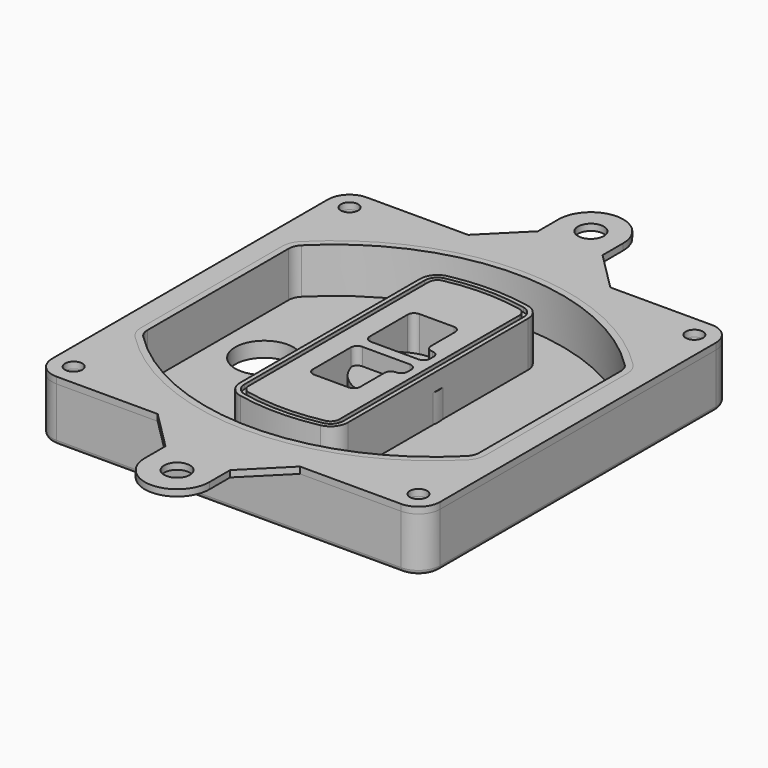
from build123d import *

# Parameters (mm, degrees)
F0_R      = 4
F1_DEPTH  = 25
F2_DEPTH  = 3
F3_DEPTH  = 18
F5_DEPTH  = 21
F6_DEPTH  = 2
F8_DEPTH  = 20
F9_DEPTH  = 16
F10_DEPTH = 25
F7_R      = 6
F7_R_2    = 4
F11_DEPTH = 6
F13_DEPTH = 9
F15_R     = 2
F16_R     = 4
F16_R_2   = 6
F17_DEPTH = 3


# Not quite as in the source:
# - a feature of the source that left no trace in its solid (it failed there, or was rolled back) is left out
# - a feature names something its author has since deleted; it is built from what else it names


with BuildPart() as f1:
    # F0 (on Top) → F1 (new body)
    with BuildSketch(Plane.XY):
        with BuildLine():
            ThreePointArc((-90, -80), (-87.0710678119, -87.0710678119), (-80, -90))
            Line((-80, -90), (80, -90))
            ThreePointArc((80, -90), (87.0710678119, -87.0710678119), (90, -80))
            Line((90, -80), (90, 80))
            ThreePointArc((90, 80), (87.0710678119, 87.0710678119), (80, 90))
            Line((80, 90), (-80, 90))
            ThreePointArc((-80, 90), (-87.0710678119, 87.0710678119), (-90, 80))
            Line((-90, 80), (-90, -80))
        make_face()
        with Locations((-80, -80)):
            Circle(F0_R, mode=Mode.SUBTRACT)
        with Locations((80, -80)):
            Circle(F0_R, mode=Mode.SUBTRACT)
        with BuildLine():
            ThreePointArc((-84, 40.977524478), (-82.9361107095, 46.3307515151), (-79.9061371841, 50.8703727074))
            ThreePointArc((-79.9061371841, 50.8703727074), (0, 84), (79.9061371841, 50.8703727074))
            ThreePointArc((79.9061371841, 50.8703727074), (82.9361107095, 46.3307515151), (84, 40.977524478))
            Line((84, 40.977524478), (84, -40.977524478))
            ThreePointArc((84, -40.977524478), (82.9361107095, -46.3307515151), (79.9061371841, -50.8703727074))
            ThreePointArc((79.9061371841, -50.8703727074), (0, -84), (-79.9061371841, -50.8703727074))
            ThreePointArc((-79.9061371841, -50.8703727074), (-82.9361107095, -46.3307515151), (-84, -40.977524478))
            Line((-84, -40.977524478), (-84, 40.977524478))
        make_face(mode=Mode.SUBTRACT)
        with Locations((-80, 80)):
            Circle(F0_R, mode=Mode.SUBTRACT)
        with Locations((80, 80)):
            Circle(F0_R, mode=Mode.SUBTRACT)
        with BuildLine():
            ThreePointArc((79.9061371841, 50.8703727074), (0, 84), (-79.9061371841, 50.8703727074))
            ThreePointArc((-79.9061371841, 50.8703727074), (-82.9361107095, 46.3307515151), (-84, 40.977524478))
            Line((-84, 40.977524478), (-84, -40.977524478))
            ThreePointArc((-84, -40.977524478), (-82.9361107095, -46.3307515151), (-79.9061371841, -50.8703727074))
            ThreePointArc((-79.9061371841, -50.8703727074), (0, -84), (79.9061371841, -50.8703727074))
            ThreePointArc((79.9061371841, -50.8703727074), (82.9361107095, -46.3307515151), (84, -40.977524478))
            Line((84, -40.977524478), (84, 40.977524478))
            ThreePointArc((84, 40.977524478), (82.9361107095, 46.3307515151), (79.9061371841, 50.8703727074))
        make_face()
        with BuildLine():
            Line((-80, -40.977524478), (-80, 40.977524478))
            ThreePointArc((-80, 40.977524478), (-79.2400790782, 44.801258076), (-77.0758122744, 48.0438446418))
            ThreePointArc((-77.0758122744, 48.0438446418), (0, 80), (77.0758122744, 48.0438446418))
            ThreePointArc((77.0758122744, 48.0438446418), (79.2400790782, 44.801258076), (80, 40.977524478))
            Line((80, 40.977524478), (80, -40.977524478))
            ThreePointArc((80, -40.977524478), (79.2400790782, -44.801258076), (77.0758122744, -48.0438446418))
            ThreePointArc((77.0758122744, -48.0438446418), (0, -80), (-77.0758122744, -48.0438446418))
            ThreePointArc((-77.0758122744, -48.0438446418), (-79.2400790782, -44.801258076), (-80, -40.977524478))
        make_face(mode=Mode.SUBTRACT)
        with BuildLine():
            ThreePointArc((-77.0758122744, 48.0438446418), (-79.2400790782, 44.801258076), (-80, 40.977524478))
            Line((-80, 40.977524478), (-80, -40.977524478))
            ThreePointArc((-80, -40.977524478), (-79.2400790782, -44.801258076), (-77.0758122744, -48.0438446418))
            ThreePointArc((-77.0758122744, -48.0438446418), (0, -80), (77.0758122744, -48.0438446418))
            ThreePointArc((77.0758122744, -48.0438446418), (79.2400790782, -44.801258076), (80, -40.977524478))
            Line((80, -40.977524478), (80, 40.977524478))
            ThreePointArc((80, 40.977524478), (79.2400790782, 44.801258076), (77.0758122744, 48.0438446418))
            ThreePointArc((77.0758122744, 48.0438446418), (0, 80), (-77.0758122744, 48.0438446418))
        make_face()
        with BuildLine():
            ThreePointArc((74.9530685921, 45.9239485927), (76.4680553548, 43.6541379966), (77, 40.977524478))
            Line((77, 40.977524478), (77, -40.977524478))
            ThreePointArc((77, -40.977524478), (76.4680553548, -43.6541379966), (74.9530685921, -45.9239485927))
            ThreePointArc((74.9530685921, -45.9239485927), (0, -77), (-74.9530685921, -45.9239485927))
            ThreePointArc((-74.9530685921, -45.9239485927), (-76.4680553548, -43.6541379966), (-77, -40.977524478))
            Line((-77, -40.977524478), (-77, 40.977524478))
            ThreePointArc((-77, 40.977524478), (-76.4680553548, 43.6541379966), (-74.9530685921, 45.9239485927))
            ThreePointArc((-74.9530685921, 45.9239485927), (0, 77), (74.9530685921, 45.9239485927))
        make_face(mode=Mode.SUBTRACT)
        with BuildLine():
            Line((77, -40.977524478), (77, 40.977524478))
            ThreePointArc((77, 40.977524478), (76.4680553548, 43.6541379966), (74.9530685921, 45.9239485927))
            ThreePointArc((74.9530685921, 45.9239485927), (0, 77), (-74.9530685921, 45.9239485927))
            ThreePointArc((-74.9530685921, 45.9239485927), (-76.4680553548, 43.6541379966), (-77, 40.977524478))
            Line((-77, 40.977524478), (-77, -40.977524478))
            ThreePointArc((-77, -40.977524478), (-76.4680553548, -43.6541379966), (-74.9530685921, -45.9239485927))
            ThreePointArc((-74.9530685921, -45.9239485927), (0, -77), (74.9530685921, -45.9239485927))
            ThreePointArc((74.9530685921, -45.9239485927), (76.4680553548, -43.6541379966), (77, -40.977524478))
        make_face()
    extrude(amount=-F1_DEPTH)

    # F0 (on Top) → F2 (join)
    with BuildSketch(Plane.XY):
        with BuildLine():
            ThreePointArc((-77.0758122744, 48.0438446418), (-79.2400790782, 44.801258076), (-80, 40.977524478))
            Line((-80, 40.977524478), (-80, -40.977524478))
            ThreePointArc((-80, -40.977524478), (-79.2400790782, -44.801258076), (-77.0758122744, -48.0438446418))
            ThreePointArc((-77.0758122744, -48.0438446418), (0, -80), (77.0758122744, -48.0438446418))
            ThreePointArc((77.0758122744, -48.0438446418), (79.2400790782, -44.801258076), (80, -40.977524478))
            Line((80, -40.977524478), (80, 40.977524478))
            ThreePointArc((80, 40.977524478), (79.2400790782, 44.801258076), (77.0758122744, 48.0438446418))
            ThreePointArc((77.0758122744, 48.0438446418), (0, 80), (-77.0758122744, 48.0438446418))
        make_face()
        with BuildLine():
            ThreePointArc((74.9530685921, 45.9239485927), (76.4680553548, 43.6541379966), (77, 40.977524478))
            Line((77, 40.977524478), (77, -40.977524478))
            ThreePointArc((77, -40.977524478), (76.4680553548, -43.6541379966), (74.9530685921, -45.9239485927))
            ThreePointArc((74.9530685921, -45.9239485927), (0, -77), (-74.9530685921, -45.9239485927))
            ThreePointArc((-74.9530685921, -45.9239485927), (-76.4680553548, -43.6541379966), (-77, -40.977524478))
            Line((-77, -40.977524478), (-77, 40.977524478))
            ThreePointArc((-77, 40.977524478), (-76.4680553548, 43.6541379966), (-74.9530685921, 45.9239485927))
            ThreePointArc((-74.9530685921, 45.9239485927), (0, 77), (74.9530685921, 45.9239485927))
        make_face(mode=Mode.SUBTRACT)
    extrude(amount=F2_DEPTH)

    # F0 (on Top) → F3 (cut)
    with BuildSketch(Plane.XY):
        with BuildLine():
            Line((77, -40.977524478), (77, 40.977524478))
            ThreePointArc((77, 40.977524478), (76.4680553548, 43.6541379966), (74.9530685921, 45.9239485927))
            ThreePointArc((74.9530685921, 45.9239485927), (0, 77), (-74.9530685921, 45.9239485927))
            ThreePointArc((-74.9530685921, 45.9239485927), (-76.4680553548, 43.6541379966), (-77, 40.977524478))
            Line((-77, 40.977524478), (-77, -40.977524478))
            ThreePointArc((-77, -40.977524478), (-76.4680553548, -43.6541379966), (-74.9530685921, -45.9239485927))
            ThreePointArc((-74.9530685921, -45.9239485927), (0, -77), (74.9530685921, -45.9239485927))
            ThreePointArc((74.9530685921, -45.9239485927), (76.4680553548, -43.6541379966), (77, -40.977524478))
        make_face()
    extrude(amount=-F3_DEPTH, mode=Mode.SUBTRACT)

    # F4 (on face) → F5 (join, through all)
    with BuildSketch(Plane.XY.offset(3)):
        with BuildLine():
            ThreePointArc((-25, -52.2388355719), (-23.2096587819, -57.2826573186), (-18.6399655469, -60.0689385728))
            ThreePointArc((-18.6399655469, -60.0689385728), (0, -62), (18.6399655469, -60.0689385728))
            ThreePointArc((18.6399655469, -60.0689385728), (23.2096587819, -57.2826573186), (25, -52.2388355719))
            Line((25, -52.2388355719), (25, 52.2388355719))
            ThreePointArc((25, 52.2388355719), (23.2096587819, 57.2826573186), (18.6399655469, 60.0689385728))
            ThreePointArc((18.6399655469, 60.0689385728), (0, 62), (-18.6399655469, 60.0689385728))
            ThreePointArc((-18.6399655469, 60.0689385728), (-23.2096587819, 57.2826573186), (-25, 52.2388355719))
            Line((-25, 52.2388355719), (-25, -52.2388355719))
        make_face()
        with BuildLine():
            ThreePointArc((18.2299741602, 58.1114128226), (21.6572440864, 56.0217018819), (23, 52.2388355719))
            Line((23, 52.2388355719), (23, -52.2388355719))
            ThreePointArc((23, -52.2388355719), (21.6572440864, -56.0217018819), (18.2299741602, -58.1114128226))
            ThreePointArc((18.2299741602, -58.1114128226), (0, -60), (-18.2299741602, -58.1114128226))
            ThreePointArc((-18.2299741602, -58.1114128226), (-21.6572440864, -56.0217018819), (-23, -52.2388355719))
            Line((-23, -52.2388355719), (-23, 52.2388355719))
            ThreePointArc((-23, 52.2388355719), (-21.6572440864, 56.0217018819), (-18.2299741602, 58.1114128226))
            ThreePointArc((-18.2299741602, 58.1114128226), (0, 60), (18.2299741602, 58.1114128226))
        make_face(mode=Mode.SUBTRACT)
        with BuildLine():
            Line((23, -52.2388355719), (23, 52.2388355719))
            ThreePointArc((23, 52.2388355719), (21.6572440864, 56.0217018819), (18.2299741602, 58.1114128226))
            ThreePointArc((18.2299741602, 58.1114128226), (0, 60), (-18.2299741602, 58.1114128226))
            ThreePointArc((-18.2299741602, 58.1114128226), (-21.6572440864, 56.0217018819), (-23, 52.2388355719))
            Line((-23, 52.2388355719), (-23, -52.2388355719))
            ThreePointArc((-23, -52.2388355719), (-21.6572440864, -56.0217018819), (-18.2299741602, -58.1114128226))
            ThreePointArc((-18.2299741602, -58.1114128226), (0, -60), (18.2299741602, -58.1114128226))
            ThreePointArc((18.2299741602, -58.1114128226), (21.6572440864, -56.0217018819), (23, -52.2388355719))
        make_face()
        with BuildLine():
            ThreePointArc((17.8199827735, 56.1538870724), (20.104829391, 54.7607464453), (21, 52.2388355719))
            Line((21, 52.2388355719), (21, -52.2388355719))
            ThreePointArc((21, -52.2388355719), (20.104829391, -54.7607464453), (17.8199827735, -56.1538870724))
            ThreePointArc((17.8199827735, -56.1538870724), (0, -58), (-17.8199827735, -56.1538870724))
            ThreePointArc((-17.8199827735, -56.1538870724), (-20.104829391, -54.7607464453), (-21, -52.2388355719))
            Line((-21, -52.2388355719), (-21, 52.2388355719))
            ThreePointArc((-21, 52.2388355719), (-20.104829391, 54.7607464453), (-17.8199827735, 56.1538870724))
            ThreePointArc((-17.8199827735, 56.1538870724), (0, 58), (17.8199827735, 56.1538870724))
        make_face(mode=Mode.SUBTRACT)
        with BuildLine():
            Line((21, -52.2388355719), (21, 52.2388355719))
            ThreePointArc((21, 52.2388355719), (20.104829391, 54.7607464453), (17.8199827735, 56.1538870724))
            ThreePointArc((17.8199827735, 56.1538870724), (0, 58), (-17.8199827735, 56.1538870724))
            ThreePointArc((-17.8199827735, 56.1538870724), (-20.104829391, 54.7607464453), (-21, 52.2388355719))
            Line((-21, 52.2388355719), (-21, -52.2388355719))
            ThreePointArc((-21, -52.2388355719), (-20.104829391, -54.7607464453), (-17.8199827735, -56.1538870724))
            ThreePointArc((-17.8199827735, -56.1538870724), (0, -58), (17.8199827735, -56.1538870724))
            ThreePointArc((17.8199827735, -56.1538870724), (20.104829391, -54.7607464453), (21, -52.2388355719))
        make_face()
        with BuildLine():
            Line((-8, -2.5), (14, -2.5))
            ThreePointArc((14, -2.5), (16.1213203436, -3.3786796564), (17, -5.5))
            Line((17, -5.5), (17, -7.5))
            ThreePointArc((17, -7.5), (16.1213203436, -9.6213203436), (14, -10.5))
            ThreePointArc((14, -10.5), (11.8786796564, -11.3786796564), (11, -13.5))
            Line((11, -13.5), (11, -27.5))
            ThreePointArc((11, -27.5), (10.1213203436, -29.6213203436), (8, -30.5))
            Line((8, -30.5), (-8, -30.5))
            ThreePointArc((-8, -30.5), (-10.1213203436, -29.6213203436), (-11, -27.5))
            Line((-11, -27.5), (-11, -5.5))
            ThreePointArc((-11, -5.5), (-10.1213203436, -3.3786796564), (-8, -2.5))
        make_face(mode=Mode.SUBTRACT)
        with BuildLine():
            ThreePointArc((-8, 2.5), (-10.1213203436, 3.3786796564), (-11, 5.5))
            Line((-11, 5.5), (-11, 27.5))
            ThreePointArc((-11, 27.5), (-10.1213203436, 29.6213203436), (-8, 30.5))
            Line((-8, 30.5), (8, 30.5))
            ThreePointArc((8, 30.5), (10.1213203436, 29.6213203436), (11, 27.5))
            Line((11, 27.5), (11, 13.5))
            ThreePointArc((11, 13.5), (11.8786796564, 11.3786796564), (14, 10.5))
            ThreePointArc((14, 10.5), (16.1213203436, 9.6213203436), (17, 7.5))
            Line((17, 7.5), (17, 5.5))
            ThreePointArc((17, 5.5), (16.1213203436, 3.3786796564), (14, 2.5))
            Line((14, 2.5), (-8, 2.5))
        make_face(mode=Mode.SUBTRACT)
    extrude(amount=-F5_DEPTH)

    # F4 (on face) → F6 (cut)
    with BuildSketch(Plane.XY.offset(3)):
        with BuildLine():
            Line((23, -52.2388355719), (23, 52.2388355719))
            ThreePointArc((23, 52.2388355719), (21.6572440864, 56.0217018819), (18.2299741602, 58.1114128226))
            ThreePointArc((18.2299741602, 58.1114128226), (0, 60), (-18.2299741602, 58.1114128226))
            ThreePointArc((-18.2299741602, 58.1114128226), (-21.6572440864, 56.0217018819), (-23, 52.2388355719))
            Line((-23, 52.2388355719), (-23, -52.2388355719))
            ThreePointArc((-23, -52.2388355719), (-21.6572440864, -56.0217018819), (-18.2299741602, -58.1114128226))
            ThreePointArc((-18.2299741602, -58.1114128226), (0, -60), (18.2299741602, -58.1114128226))
            ThreePointArc((18.2299741602, -58.1114128226), (21.6572440864, -56.0217018819), (23, -52.2388355719))
        make_face()
        with BuildLine():
            ThreePointArc((17.8199827735, 56.1538870724), (20.104829391, 54.7607464453), (21, 52.2388355719))
            Line((21, 52.2388355719), (21, -52.2388355719))
            ThreePointArc((21, -52.2388355719), (20.104829391, -54.7607464453), (17.8199827735, -56.1538870724))
            ThreePointArc((17.8199827735, -56.1538870724), (0, -58), (-17.8199827735, -56.1538870724))
            ThreePointArc((-17.8199827735, -56.1538870724), (-20.104829391, -54.7607464453), (-21, -52.2388355719))
            Line((-21, -52.2388355719), (-21, 52.2388355719))
            ThreePointArc((-21, 52.2388355719), (-20.104829391, 54.7607464453), (-17.8199827735, 56.1538870724))
            ThreePointArc((-17.8199827735, 56.1538870724), (0, 58), (17.8199827735, 56.1538870724))
        make_face(mode=Mode.SUBTRACT)
    extrude(amount=-F6_DEPTH, mode=Mode.SUBTRACT)

    # F7 (on face) → F8 (join)
    with BuildSketch(Plane(origin=(0, 0, -25), x_dir=(1, 0, 0), z_dir=(0, 0, -1))):
        with BuildLine():
            ThreePointArc((-6.71157564, 0), (6.7567035675, 13.4682792075), (20.224982775, 0))
            Line((20.224982775, 0), (25.224982775, 0))
            ThreePointArc((25.224982775, 0), (6.7567035675, 18.4682792075), (-11.71157564, 0))
            Line((-11.71157564, 0), (-6.71157564, 0))
        make_face()
        with BuildLine():
            Line((-6.71157564, 0), (20.224982775, 0))
            ThreePointArc((20.224982775, 0), (6.7567035675, 13.4682792075), (-6.71157564, 0))
        make_face()
        with BuildLine():
            ThreePointArc((-6.71157564, 0), (6.7567035675, -13.4682792075), (20.224982775, 0))
            Line((20.224982775, 0), (-6.71157564, 0))
        make_face()
        with BuildLine():
            Line((25.224982775, 0), (20.224982775, 0))
            ThreePointArc((20.224982775, 0), (6.7567035675, -13.4682792075), (-6.71157564, 0))
            Line((-6.71157564, 0), (-11.71157564, 0))
            ThreePointArc((-11.71157564, 0), (6.7567035675, -18.4682792075), (25.224982775, 0))
        make_face()
    extrude(amount=-F8_DEPTH)

    # F7 (on face) → F9 (cut)
    with BuildSketch(Plane(origin=(0, 0, -25), x_dir=(1, 0, 0), z_dir=(0, 0, -1))):
        with BuildLine():
            Line((-6.71157564, 0), (20.224982775, 0))
            ThreePointArc((20.224982775, 0), (6.7567035675, 13.4682792075), (-6.71157564, 0))
        make_face()
        with BuildLine():
            ThreePointArc((-6.71157564, 0), (6.7567035675, -13.4682792075), (20.224982775, 0))
            Line((20.224982775, 0), (-6.71157564, 0))
        make_face()
    extrude(amount=-F9_DEPTH, mode=Mode.SUBTRACT)

    # F7 (on face) → F10 (cut)
    with BuildSketch(Plane(origin=(0, 0, -25), x_dir=(1, 0, 0), z_dir=(0, 0, -1))):
        with BuildLine():
            Line((-69.0318229325, 0), (-42.0952645175, 0))
            ThreePointArc((-42.0952645175, 0), (-55.563543725, 13.4682792075), (-69.0318229325, 0))
        make_face()
        with BuildLine():
            ThreePointArc((-69.0318229325, 0), (-55.563543725, -13.4682792075), (-42.0952645175, 0))
            Line((-42.0952645175, 0), (-69.0318229325, 0))
        make_face()
    extrude(amount=-F10_DEPTH, mode=Mode.SUBTRACT)

    # F7 (on face) → F11 (cut)
    with BuildSketch(Plane(origin=(0, 0, -25), x_dir=(1, 0, 0), z_dir=(0, 0, -1))):
        with Locations((80, -80)):
            Circle(F7_R)
        with Locations((80, -80)):
            Circle(F7_R_2, mode=Mode.SUBTRACT)
        with Locations((-80, -80)):
            Circle(F7_R)
        with Locations((-80, -80)):
            Circle(F7_R_2, mode=Mode.SUBTRACT)
        with Locations((-80, 80)):
            Circle(F7_R)
        with Locations((-80, 80)):
            Circle(F7_R_2, mode=Mode.SUBTRACT)
        with Locations((80, 80)):
            Circle(F7_R)
        with Locations((80, 80)):
            Circle(F7_R_2, mode=Mode.SUBTRACT)
    extrude(amount=-F11_DEPTH, mode=Mode.SUBTRACT)

    # F12 (on face) → F13 (cut, through all)
    with BuildSketch(Plane(origin=(0, 0, -9), x_dir=(1, 0, 0), z_dir=(0, 0, -1))):
        with BuildLine():
            ThreePointArc((20.224982775, 0), (20.1663399806, 1.2554664788), (19.9909222755, 2.5))
            Line((19.9909222755, 2.5), (14, 2.5))
            ThreePointArc((14, 2.5), (16.1213203436, 3.3786796564), (17, 5.5))
            Line((17, 5.5), (17, 7.5))
            ThreePointArc((17, 7.5), (16.1213203436, 9.6213203436), (14, 10.5))
            ThreePointArc((14, 10.5), (12.1627255951, 11.1284134507), (11.0951631559, 12.750384826))
            ThreePointArc((11.0951631559, 12.750384826), (11.0476113807, 12.7664660322), (11, 12.7823698976))
            Line((11, 12.7823698976), (11, -12.7823698976))
            ThreePointArc((11, -12.7823698976), (11.0476113807, -12.7664660322), (11.0951631559, -12.750384826))
            ThreePointArc((11.0951631559, -12.750384826), (12.1627255951, -11.1284134507), (14, -10.5))
            ThreePointArc((14, -10.5), (16.1213203436, -9.6213203436), (17, -7.5))
            Line((17, -7.5), (17, -5.5))
            ThreePointArc((17, -5.5), (16.1213203436, -3.3786796564), (14, -2.5))
            Line((14, -2.5), (19.9909222755, -2.5))
            ThreePointArc((19.9909222755, -2.5), (20.1663399806, -1.2554664788), (20.224982775, 0))
        make_face()
    extrude(amount=F13_DEPTH, mode=Mode.SUBTRACT)

    # F15
    f15_edges = [f1.edges().sort_by_distance(p)[0] for p in [
        (0, -90, -25),
        (-87.071068, -87.071068, -25),
        (-90, 0, -25),
        (-87.071068, 87.071068, -25),
        (87.071068, -87.071068, -25),
        (0, 90, -25),
        (90, 0, -25),
        (87.071068, 87.071068, -25),
    ]]
    fillet(f15_edges, radius=F15_R)


with BuildPart() as f17:
    # F16 (on face) → F17 (new body, through all)
    with BuildSketch(Plane.XY):
        with BuildLine():
            ThreePointArc((90, 80), (87.0710678119, 87.0710678119), (80, 90))
            Line((80, 90), (33, 90))
            Line((33, 90), (15, 108))
            Line((15, 108), (15, 120))
            ThreePointArc((15, 120), (0, 135), (-15, 120))
            Line((-15, 120), (-15, 108))
            Line((-15, 108), (-33, 90))
            Line((-33, 90), (-80, 90))
            ThreePointArc((-80, 90), (-87.0710678119, 87.0710678119), (-90, 80))
            Line((-90, 80), (-90, -80))
            ThreePointArc((-90, -80), (-87.0710678119, -87.0710678119), (-80, -90))
            Line((-80, -90), (-33, -90))
            Line((-33, -90), (-15, -108))
            Line((-15, -108), (-15, -120))
            ThreePointArc((-15, -120), (0, -135), (15, -120))
            Line((15, -120), (15, -108))
            Line((15, -108), (33, -90))
            Line((33, -90), (80, -90))
            ThreePointArc((80, -90), (87.0710678119, -87.0710678119), (90, -80))
            Line((90, -80), (90, 80))
        make_face()
        with Locations((-80, -80)):
            Circle(F16_R, mode=Mode.SUBTRACT)
        with Locations((0, -120)):
            Circle(F16_R_2, mode=Mode.SUBTRACT)
        with Locations((80, -80)):
            Circle(F16_R, mode=Mode.SUBTRACT)
        with Locations((-80, 80)):
            Circle(F16_R, mode=Mode.SUBTRACT)
        with BuildLine():
            ThreePointArc((77.0758122744, -48.0438446418), (0, -80), (-77.0758122744, -48.0438446418))
            ThreePointArc((-77.0758122744, -48.0438446418), (-79.2400790782, -44.801258076), (-80, -40.977524478))
            Line((-80, -40.977524478), (-80, 40.977524478))
            ThreePointArc((-80, 40.977524478), (-79.2400790782, 44.801258076), (-77.0758122744, 48.0438446418))
            ThreePointArc((-77.0758122744, 48.0438446418), (0, 80), (77.0758122744, 48.0438446418))
            ThreePointArc((77.0758122744, 48.0438446418), (79.2400790782, 44.801258076), (80, 40.977524478))
            Line((80, 40.977524478), (80, -40.977524478))
            ThreePointArc((80, -40.977524478), (79.2400790782, -44.801258076), (77.0758122744, -48.0438446418))
        make_face(mode=Mode.SUBTRACT)
        with Locations((0, 120)):
            Circle(F16_R_2, mode=Mode.SUBTRACT)
        with Locations((80, 80)):
            Circle(F16_R, mode=Mode.SUBTRACT)
    extrude(amount=F17_DEPTH)


solid = Compound([f1.part, f17.part])
